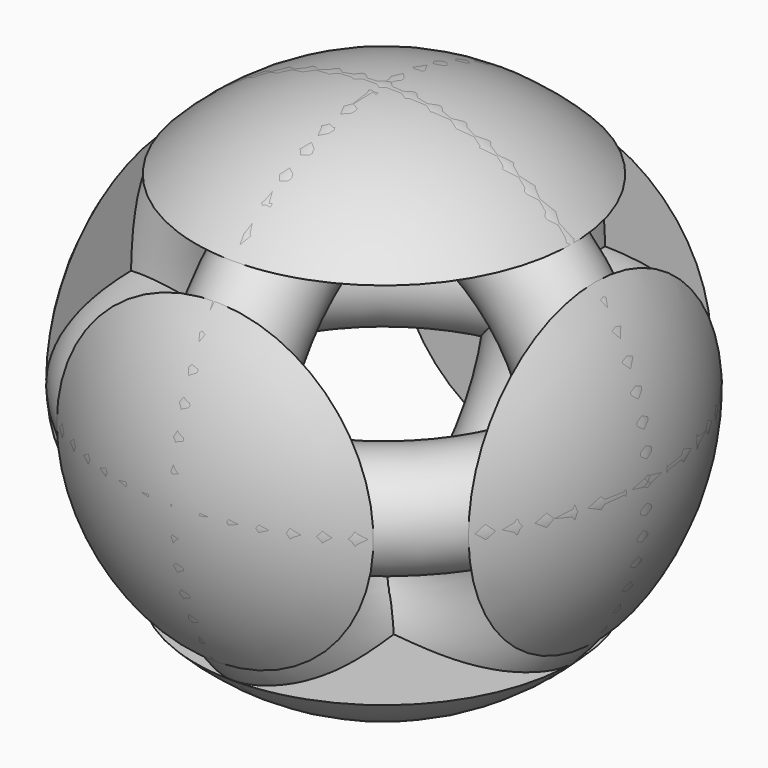
from build123d import *
from build123d import SkipClean  # not in build123d's __all__

# Parameters (mm, degrees)
F2_W     = 20.32
F2_H     = 20.32
F3_DEPTH = 8.89
F4_R     = 2.54
F6_R     = 2.54
F8_R     = 2.54


with BuildPart() as f1:
    # F0 (on Top) → F1 (revolve)
    with BuildSketch(Plane.XY):
        with BuildLine():
            Line((0, -12.7), (0, 12.7))
            ThreePointArc((0, 12.7), (-12.7, 0), (0, -12.7))
        make_face()
    revolve(axis=Axis((0, 0, 0), (0, -1, 0)))

    # F2 (on Top) → F3 (cut, symmetric)
    with BuildSketch(Plane.XY):
        Rectangle(F2_W, F2_H)
    with SkipClean():  # cleaning this boolean's faces spoils the solid; the shape is the same uncleaned
        extrude(amount=F3_DEPTH, both=True, mode=Mode.SUBTRACT)


with BuildPart() as f5:
    # F4 (on Top) → F5 (revolve)
    with BuildSketch(Plane.XY):
        with Locations((10.16, 0)):
            Circle(F4_R)
    revolve(axis=Axis((0, -5.3515611752, 0), (0, -1, 0)))


with BuildPart() as f7:
    # F6 (on Top) → F7 (revolve)
    with BuildSketch(Plane.XY):
        with Locations((0, 10.16)):
            Circle(F6_R)
    revolve(axis=Axis((7.3015755042, 0, 0), (1, 0, 0)))


with BuildPart() as f9:
    # F8 (on Right) → F9 (revolve)
    with BuildSketch(Plane.YZ):
        with Locations((10.16, 0)):
            Circle(F8_R)
    revolve(axis=Axis((0, 0, -7.2491783649), (0, 0, -1)))


solid = Compound([f1.part, f5.part, f7.part, f9.part])
